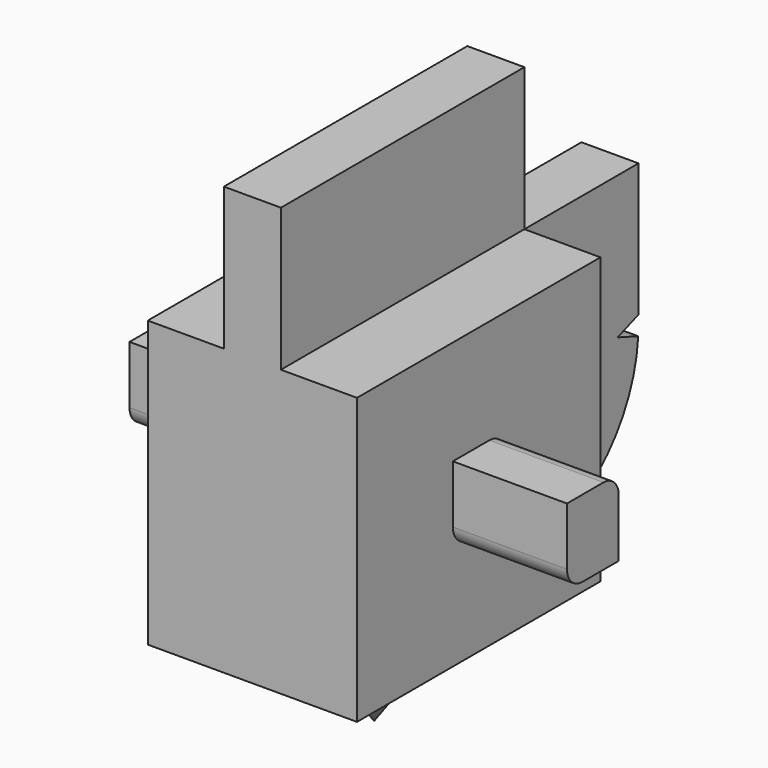
from build123d import *

# Parameters (mm, degrees)
F0_W      = 20.32
F0_H      = 19.05
F1_DEPTH  = 13.97
F3_START  = -6.985
F2_W      = 29.21
F2_H      = 4.318
F3_DEPTH  = 5.1308
F7_W      = 20.32
F7_H      = 9.525
F8_DEPTH  = 1.905
F9_DEPTH  = 9.525
F10_R     = 1.27
F12_DEPTH = 25.4


with BuildPart() as f1:
    # F0 (on Right) → F1 (new body)
    with BuildSketch(Plane.YZ):
        with Locations((10.16, -9.525)):
            Rectangle(F0_W, F0_H)
    extrude(amount=F1_DEPTH)

    # F2 (on face) → F3 (join)
    with BuildSketch(Plane.XY.offset(F3_START)):
        with Locations((6.985, 10.16)):
            Rectangle(F2_W, F2_H)
    extrude(amount=-F3_DEPTH)

    # F5 (on offset) → F6 (revolve)
    with BuildSketch(Plane.YZ.offset(6.985)):
        Polygon((10.16, -19.05), (5.715, -19.05), (10.16, -25.4), align=None)
    revolve(axis=Axis((6.985, 10.16, -22.225), (0, 0, 1)))

    # F7 (on offset) → F8 (join, symmetric)
    with BuildSketch(Plane.YZ.offset(6.985)):
        with BuildLine():
            ThreePointArc((20.32, -19.05), (27.0551920908, -16.2601920908), (29.845, -9.525))
            Line((29.845, -9.525), (20.32, -9.525))
            Line((20.32, -9.525), (20.32, -19.05))
        make_face()
        with Locations((10.16, 4.7625)):
            Rectangle(F7_W, F7_H)
    extrude(amount=F8_DEPTH, both=True)

    # F9 (add, through all): a face of the model
    f9_faces = [f1.faces().sort_by_distance(p)[0] for p in [
        (6.985, 25.0825, -9.525),
    ]]
    extrude(f9_faces, amount=F9_DEPTH)

    # F10
    f10_edges = [f1.edges().sort_by_distance(p)[0] for p in [
        (17.78, 8.001, -12.1158),
        (17.78, 12.319, -6.985),
        (-3.81, 8.001, -12.1158),
        (-3.81, 12.319, -6.985),
    ]]
    fillet(f10_edges, radius=F10_R)

    # F11 (on offset) → F12 (cut, symmetric)
    with BuildSketch(Plane.YZ.offset(6.985)):
        Polygon((29.845, -10.16), (29.845, -8.89), (28.1003518386, -9.525), align=None)
    extrude(amount=F12_DEPTH, both=True, mode=Mode.SUBTRACT)


solid = f1.part
